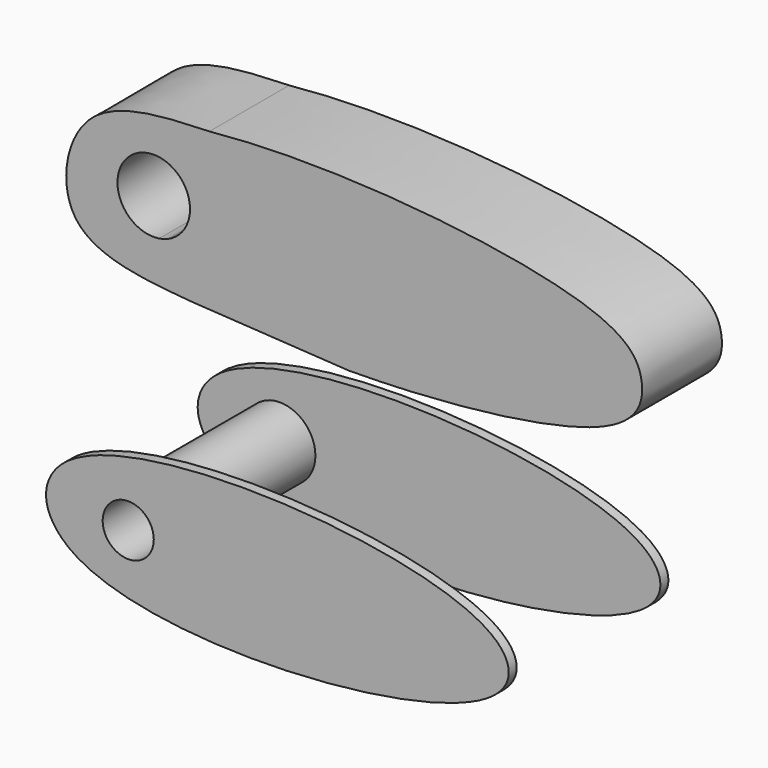
from build123d import *

# Parameters (mm, degrees)
F1_DEPTH = 25.4
F0_R     = 6.5031313052
F2_DEPTH = 50.8
F3_T     = -2.54


with BuildPart() as f1:
    # F0 (on Front) → F1 (new body)
    with BuildSketch(Plane.XZ):
        with BuildLine():
            add(Edge.make_bspline(
                [(-37.3016794588, 50.3096369225), (-49.5612955383, 49.874227496), (-61.8209134363, 49.438818675), (-68.4245601296, 42.440533638)],
                knots=[0, 0, 0, 0, 0.3537381003, 0.3537381003, 0.3537381003, 0.3537381003], degree=3))
            add(Edge.make_bspline(
                [(-68.4245601296, 42.440533638), (-61.3210683551, 46.5254168024), (-50.2032400778, 49.0288539057), (-37.3016794588, 50.3096369225)],
                knots=[0, 0, 0, 0, 0.0881515709, 0.0881515709, 0.0881515709, 0.0881515709], degree=3))
        make_face()
        with BuildLine():
            add(Edge.make_bspline(
                [(-68.4245601296, 42.440533638), (-61.3210683551, 46.5254168024), (-50.2032400778, 49.0288539057), (-37.3016794588, 50.3096369225)],
                knots=[0, 0, 0, 0, 0.0881515709, 0.0881515709, 0.0881515709, 0.0881515709], degree=3))
            add(Edge.make_bspline(
                [(-68.4245601296, 42.440533638), (-73.9803374412, 36.552739358), (-75.5327128562, 26.0196189357), (-71.4560225831, 19.9210644105)],
                knots=[0.3537381003, 0.3537381003, 0.3537381003, 0.3537381003, 0.651344893, 0.651344893, 0.651344893, 0.651344893], degree=3))
            add(Edge.make_bspline(
                [(-41.6765425697, 10.6598649355), (-54.6326703325, 12.5398531998), (-65.3812225897, 15.5646773895), (-71.4560225936, 19.9210644005)],
                knots=[0.7802465657, 0.7802465657, 0.7802465657, 0.7802465657, 0.8673123975, 0.8673123975, 0.8673123975, 0.8673123975], degree=3))
            add(Edge.make_bspline(
                [(-1.7571478697, 8.2351713018), (-15.0636128696, 9.0434025239), (-28.3700775698, 9.8516337134), (-41.6765425697, 10.6598649355)],
                knots=[0, 0, 0, 0, 39.9929645366, 39.9929645366, 39.9929645366, 39.9929645366], degree=3))
            add(Edge.make_bspline(
                [(-37.3016794588, 50.3096369225), (-4.07805523, 53.6078622243), (64.2631466821, 46.3118000236), (74.7357462917, 30.6114232797), (70.0766156824, 13.9623902843), (24.8192939413, 8.3937822593), (-1.7571478697, 8.2351713018)],
                knots=[0.0881515709, 0.0881515709, 0.0881515709, 0.0881515709, 0.3151562532, 0.4325012261, 0.5442294678, 0.6992219052, 0.6992219052, 0.6992219052, 0.6992219052], degree=3))
        make_face()
        with BuildLine():
            ThreePointArc((-50.0915318784, 22.141829717), (-58.4783217971, 37.2909738773), (-42.2426453777, 31.2712043524))
            ThreePointArc((-42.2426453777, 31.2712043524), (-43.7354082391, 26.2373704922), (-47.7310494308, 22.8311004267))
            ThreePointArc((-47.7310494308, 22.8311004267), (-48.8882430876, 22.4075361742), (-50.0915318784, 22.141829717))
        make_face(mode=Mode.SUBTRACT)
        with BuildLine():
            add(Edge.make_bspline(
                [(-41.6765425697, 10.6598649355), (-54.6326703325, 12.5398531998), (-65.3812225897, 15.5646773895), (-71.4560225936, 19.9210644005)],
                knots=[0.7802465657, 0.7802465657, 0.7802465657, 0.7802465657, 0.8673123975, 0.8673123975, 0.8673123975, 0.8673123975], degree=3))
            add(Edge.make_bspline(
                [(-71.4560225831, 19.9210644105), (-66.6800600512, 12.7764284534), (-54.1783109824, 11.718150589), (-41.6765425697, 10.6598649355)],
                knots=[0.651344893, 0.651344893, 0.651344893, 0.651344893, 1, 1, 1, 1], degree=3))
        make_face()
    extrude(amount=F1_DEPTH)


with BuildPart() as f2:
    # F0 (on Front) → F2 (new body)
    with BuildSketch(Plane.XZ):
        with BuildLine():
            add(Edge.make_bspline(
                [(-52.8341531754, -18.1888192892), (-33.8467723013, -4.9405199348), (58.1503454425, -10.0400248252), (63.6521748358, -46.6063467776), (-57.8384824747, -54.3591655746), (-61.3733754013, -24.1469960938), (-52.8341531754, -18.1888192892)],
                knots=[0, 0, 0, 0, 0.3535570474, 0.4881202407, 0.8409942784, 1, 1, 1, 1], degree=3))
        make_face()
        with Locations((-37.6492440701, -28.8522411138)):
            Circle(F0_R, mode=Mode.SUBTRACT)
    extrude(amount=F2_DEPTH)

    # F3
    f3_openings = [f2.faces().sort_by_distance(p)[0] for p in [
        (53.153874, -25.4, -37.156652),
    ]]
    offset(amount=F3_T, openings=f3_openings)


solid = Compound([f1.part, f2.part])
